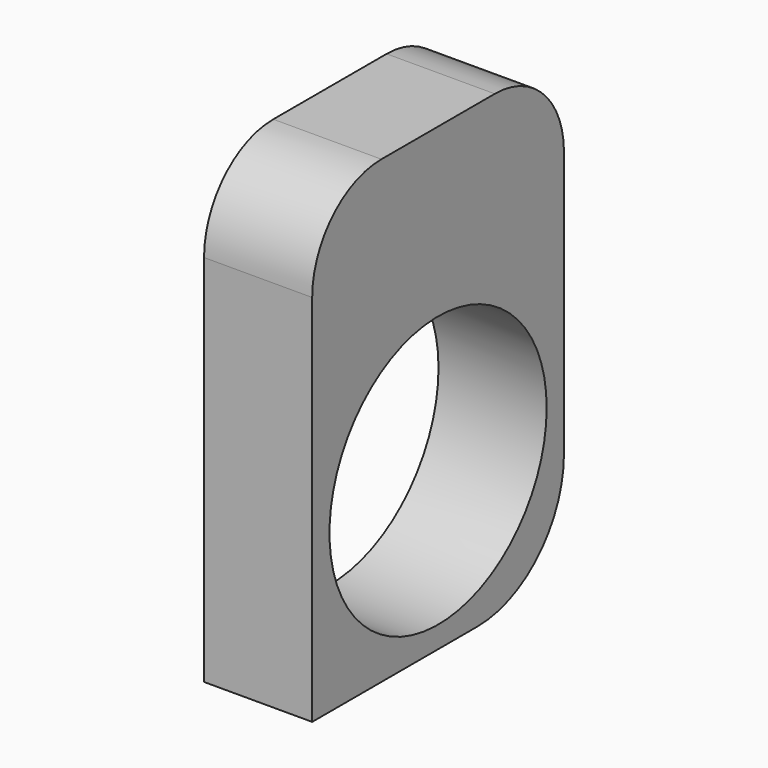
from build123d import *

# Parameters (mm, degrees)
F0_R     = 12.55
F1_DEPTH = 5
F2_DEPTH = 5
F3_R     = 10


with BuildPart() as f1:
    # F0 (on Right) → F1 (new body)
    with BuildSketch(Plane.YZ):
        with BuildLine():
            ThreePointArc((14.55, 20), (12.2068542495, 25.6568542495), (6.55, 28))
            Line((6.55, 28), (-6.55, 28))
            ThreePointArc((-6.55, 28), (-12.2068542495, 25.6568542495), (-14.55, 20))
            Line((-14.55, 20), (-14.55, -14.55))
            Line((-14.55, -14.55), (14.55, -14.55))
            Line((14.55, -14.55), (14.55, 20))
        make_face()
        Circle(F0_R, mode=Mode.SUBTRACT)
        with BuildLine():
            Line((2.8404028665, 18.7938524157), (-4.0904028665, 18.7938524157))
            ThreePointArc((-4.0904028665, 18.7938524157), (-6.8404028665, 16.0438524157), (-9.5904028665, 18.7938524157))
            ThreePointArc((-9.5904028665, 18.7938524157), (-8.8718404378, 20.6474331111), (-7.0916673072, 21.5323494818))
            Line((-7.0916673072, 21.5323494818), (6.4749272755, 22.7771208717))
            ThreePointArc((6.4749272755, 22.7771208717), (9.5365202263, 21.748670715), (10.8404028665, 18.7938524157))
            ThreePointArc((10.8404028665, 18.7938524157), (6.8404028665, 14.7938524157), (2.8404028665, 18.7938524157))
        make_face(mode=Mode.SUBTRACT)
        with BuildLine():
            ThreePointArc((-7.0916673072, 21.5323494818), (-4.9868221712, 20.825289987), (-4.0904028665, 18.7938524157))
            Line((-4.0904028665, 18.7938524157), (2.8404028665, 18.7938524157))
            ThreePointArc((2.8404028665, 18.7938524157), (3.8855845672, 21.4899697755), (6.4749272755, 22.7771208717))
            Line((6.4749272755, 22.7771208717), (-7.0916673072, 21.5323494818))
        make_face()
    extrude(amount=-F1_DEPTH)

    # F0 (on Right) → F2 (join)
    with BuildSketch(Plane.YZ):
        with BuildLine():
            ThreePointArc((14.55, 20), (12.2068542495, 25.6568542495), (6.55, 28))
            Line((6.55, 28), (-6.55, 28))
            ThreePointArc((-6.55, 28), (-12.2068542495, 25.6568542495), (-14.55, 20))
            Line((-14.55, 20), (-14.55, -14.55))
            Line((-14.55, -14.55), (14.55, -14.55))
            Line((14.55, -14.55), (14.55, 20))
        make_face()
        Circle(F0_R, mode=Mode.SUBTRACT)
        with BuildLine():
            Line((2.8404028665, 18.7938524157), (-4.0904028665, 18.7938524157))
            ThreePointArc((-4.0904028665, 18.7938524157), (-6.8404028665, 16.0438524157), (-9.5904028665, 18.7938524157))
            ThreePointArc((-9.5904028665, 18.7938524157), (-8.8718404378, 20.6474331111), (-7.0916673072, 21.5323494818))
            Line((-7.0916673072, 21.5323494818), (6.4749272755, 22.7771208717))
            ThreePointArc((6.4749272755, 22.7771208717), (9.5365202263, 21.748670715), (10.8404028665, 18.7938524157))
            ThreePointArc((10.8404028665, 18.7938524157), (6.8404028665, 14.7938524157), (2.8404028665, 18.7938524157))
        make_face(mode=Mode.SUBTRACT)
        with BuildLine():
            ThreePointArc((-9.5904028665, 18.7938524157), (-6.8404028665, 16.0438524157), (-4.0904028665, 18.7938524157))
            Line((-4.0904028665, 18.7938524157), (-9.5904028665, 18.7938524157))
        make_face()
        with BuildLine():
            Line((-9.5904028665, 18.7938524157), (-4.0904028665, 18.7938524157))
            ThreePointArc((-4.0904028665, 18.7938524157), (-4.9868221712, 20.825289987), (-7.0916673072, 21.5323494818))
            ThreePointArc((-7.0916673072, 21.5323494818), (-8.8718404378, 20.6474331111), (-9.5904028665, 18.7938524157))
        make_face()
        with BuildLine():
            ThreePointArc((-7.0916673072, 21.5323494818), (-4.9868221712, 20.825289987), (-4.0904028665, 18.7938524157))
            Line((-4.0904028665, 18.7938524157), (2.8404028665, 18.7938524157))
            ThreePointArc((2.8404028665, 18.7938524157), (3.8855845672, 21.4899697755), (6.4749272755, 22.7771208717))
            Line((6.4749272755, 22.7771208717), (-7.0916673072, 21.5323494818))
        make_face()
        with BuildLine():
            ThreePointArc((6.4749272755, 22.7771208717), (3.8855845672, 21.4899697755), (2.8404028665, 18.7938524157))
            Line((2.8404028665, 18.7938524157), (10.8404028665, 18.7938524157))
            ThreePointArc((10.8404028665, 18.7938524157), (9.5365202263, 21.748670715), (6.4749272755, 22.7771208717))
        make_face()
        with BuildLine():
            Line((10.8404028665, 18.7938524157), (2.8404028665, 18.7938524157))
            ThreePointArc((2.8404028665, 18.7938524157), (6.8404028665, 14.7938524157), (10.8404028665, 18.7938524157))
        make_face()
    extrude(amount=F2_DEPTH)

    # F3
    f3_edges = [f1.edges().sort_by_distance(p)[0] for p in [
        (0, 14.55, -14.55),
    ]]
    fillet(f3_edges, radius=F3_R)

    # F0 (on Right) → F4 (revolve, cut)
    with BuildSketch(Plane.YZ):
        with BuildLine():
            Line((-9.5904028665, 18.7938524157), (-4.0904028665, 18.7938524157))
            ThreePointArc((-4.0904028665, 18.7938524157), (-4.9868221712, 20.825289987), (-7.0916673072, 21.5323494818))
            ThreePointArc((-7.0916673072, 21.5323494818), (-8.8718404378, 20.6474331111), (-9.5904028665, 18.7938524157))
        make_face()
        with BuildLine():
            ThreePointArc((-7.0916673072, 21.5323494818), (-4.9868221712, 20.825289987), (-4.0904028665, 18.7938524157))
            Line((-4.0904028665, 18.7938524157), (2.8404028665, 18.7938524157))
            ThreePointArc((2.8404028665, 18.7938524157), (3.8855845672, 21.4899697755), (6.4749272755, 22.7771208717))
            Line((6.4749272755, 22.7771208717), (-7.0916673072, 21.5323494818))
        make_face()
        with BuildLine():
            ThreePointArc((6.4749272755, 22.7771208717), (3.8855845672, 21.4899697755), (2.8404028665, 18.7938524157))
            Line((2.8404028665, 18.7938524157), (10.8404028665, 18.7938524157))
            ThreePointArc((10.8404028665, 18.7938524157), (9.5365202263, 21.748670715), (6.4749272755, 22.7771208717))
        make_face()
    revolve(axis=Axis((0, 0.625, 18.7938524157), (0, 1, 0)), mode=Mode.SUBTRACT)


solid = f1.part
